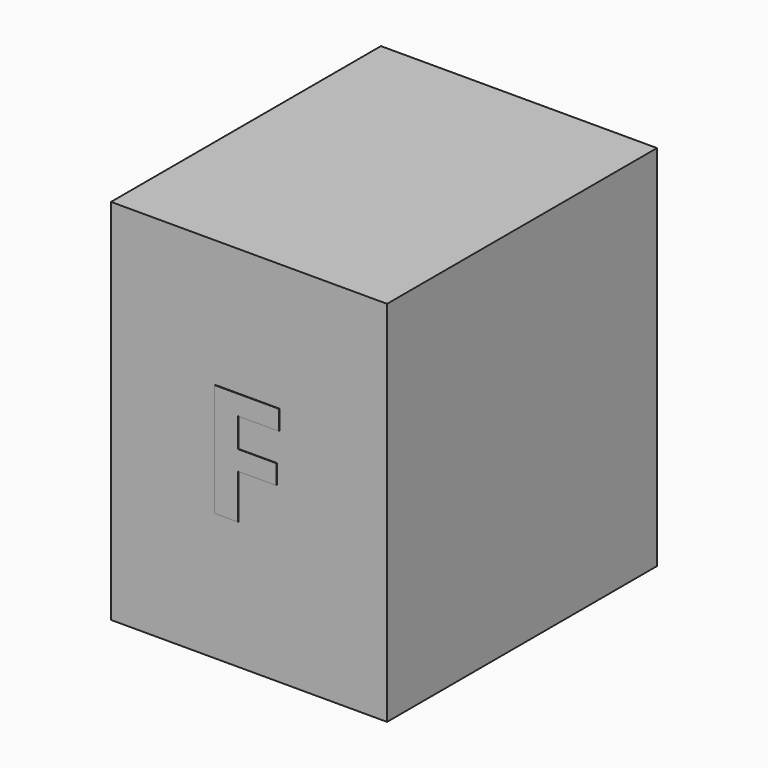
from build123d import *

# Parameters (mm, degrees)
F0_W         = 450
F0_H         = 550
F1_DEPTH     = 600
F2_TEXT_SIZE = 257.8243199322
F3_DEPTH     = 1


# Not quite as in the source:
# - Text() gives the source's letters only with a copy of the font that has no kerning and outlines rounded to 1/6400 em; it was checked with that copy


with BuildPart() as f1:
    # F0 (on Top) → F1 (new body)
    with BuildSketch(Plane.XY):
        Rectangle(F0_W, F0_H)
    extrude(amount=F1_DEPTH)

    # F2 (on face) → F3 (join)
    with BuildSketch(Plane.XZ.offset(275)):
        with Locations((-78.7984579802, 208.5310816765)):
            Text('F', F2_TEXT_SIZE, font='Open Sans', font_style=FontStyle.BOLD, text_align=(TextAlign.LEFT, TextAlign.BOTTOM))
    extrude(amount=F3_DEPTH)


solid = f1.part
